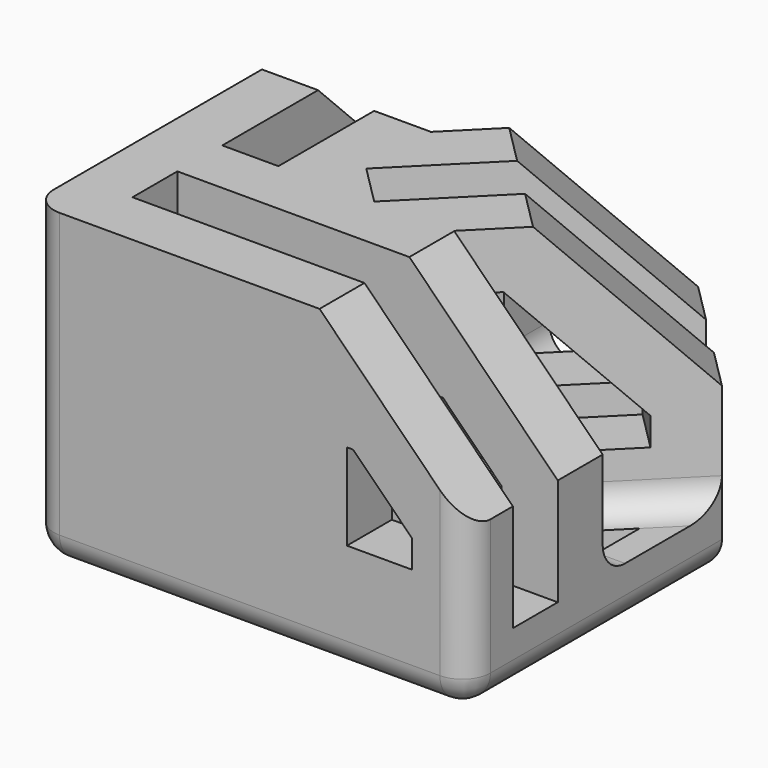
from build123d import *

# Parameters (mm, degrees)
F1_DEPTH      = 41
F3_DEPTH      = 9
F4_SIZE       = 23.8
F5_SIZE       = 23.8
F7_DEPTH      = 9
F9_DEPTH      = 28.2
F11_DEPTH     = 34.5
F13_DEPTH     = 32.2
F14_R         = 4.49999
F15_T4_DEPTH  = 56.311183182
F15_T10_DEPTH = 35.158116908
F15_T15_DEPTH = 56.311183182
F15_T21_DEPTH = 35.158116908
F15_T23_DEPTH = 61.25
F15_T25_DEPTH = 37.45
F15_T28_ANGLE = 90
F15_T30_ANGLE = 90
F15_T32_ANGLE = 90


# Not quite as in the source:
# - a fillet or chamfer that OpenCascade refuses, or shapes differently, is made with other operations: its cross-section is extruded or revolved along the edge and cut away or added
# - a fillet or chamfer is up to 0.001 mm smaller than in the source, because OpenCascade refuses the exact size


with BuildPart() as f1:
    # F0 (on Top) → F1 (new body)
    with BuildSketch(Plane.XY):
        Polygon((0, 70), (0, 0), (70, 0), (70, 9), (9, 9), (9, 18), (70, 18), (70, 27), (46.091883092, 27), (70, 50.908116908), (63.6360389693, 57.2720779386), (33.3639610307, 27), (27, 33.3639610307), (57.2720779386, 63.6360389693), (50.908116908, 70), (27, 46.091883092), (27, 70), (18, 70), (18, 27), (9, 27), (9, 70), align=None)
    extrude(amount=F1_DEPTH)

    # F2 (on face) → F3 (join)
    with BuildSketch(Plane(origin=(0, 0, 0), x_dir=(1, 0, 0), z_dir=(0, 0, -1))):
        Polygon((70, -50.908116908), (70, 0), (0, 0), (0, -70), (50.908116908, -70), align=None)
    extrude(amount=F3_DEPTH)

    # F4
    f4_edges = [f1.edges().sort_by_distance(p)[0] for p in [
        (70, 4.5, 41),
        (70, 22.5, 41),
        (22.5, 70, 41),
        (4.5, 70, 41),
    ]]
    chamfer(f4_edges, length=F4_SIZE)

    # F5
    f5_edges = [f1.edges().sort_by_distance(p)[0] for p in [
        (66.818019, 54.090097, 41),
        (54.090097, 66.818019, 41),
    ]]
    chamfer(f5_edges, length=F5_SIZE)

    # F6 (on face) → F7 (cut, through all)
    with BuildSketch(Plane.XY):
        with BuildLine():
            Line((9, 56.5), (9, 31.5))
            ThreePointArc((9, 31.5), (10.3180194847, 28.3180194847), (13.5, 27))
            ThreePointArc((13.5, 27), (16.6819805153, 28.3180194847), (18, 31.5))
            Line((18, 31.5), (18, 56.5))
            ThreePointArc((18, 56.5), (16.6819805153, 59.6819805153), (13.5, 61))
            ThreePointArc((13.5, 61), (10.3180194847, 59.6819805153), (9, 56.5))
        make_face()
        with BuildLine():
            Line((56.5, 18), (13.5, 18))
            ThreePointArc((13.5, 18), (10.3180194847, 16.6819805153), (9, 13.5))
            ThreePointArc((9, 13.5), (10.3180194847, 10.3180194847), (13.5, 9))
            Line((13.5, 9), (56.5, 9))
            ThreePointArc((56.5, 9), (59.6819805153, 10.3180194847), (61, 13.5))
            ThreePointArc((61, 13.5), (59.6819805153, 16.6819805153), (56.5, 18))
        make_face()
        with BuildLine():
            Line((47.7261363926, 54.0900974233), (30.1819805153, 36.545941546))
            ThreePointArc((30.1819805153, 36.545941546), (28.8639610307, 33.3639610307), (30.1819805153, 30.1819805153))
            ThreePointArc((30.1819805153, 30.1819805153), (33.3639610307, 28.8639610307), (36.545941546, 30.1819805153))
            Line((36.545941546, 30.1819805153), (54.0900974233, 47.7261363926))
            ThreePointArc((54.0900974233, 47.7261363926), (55.408116908, 50.908116908), (54.0900974233, 54.0900974233))
            ThreePointArc((54.0900974233, 54.0900974233), (50.908116908, 55.408116908), (47.7261363926, 54.0900974233))
        make_face()
        Polygon((40.0441558773, 65.5), (31.5, 65.5), (31.5, 56.9558441227), align=None)
        Polygon((65.5, 40.0441558773), (56.9558441227, 31.5), (65.5, 31.5), align=None)
    extrude(amount=-F7_DEPTH, mode=Mode.SUBTRACT)

    # F8 (on face) → F9 (cut)
    with BuildSketch(Plane(origin=(9.545941546, -9.545941546, 0), x_dir=(0.7071067812, 0.7071067812, 0), z_dir=(0.7071067812, -0.7071067812, 0))):
        Polygon((56.1837661841, 32), (56.1837661841, 9), (76.4949493661, 9), (76.4949493661, 13.4720779386), (57.9670273048, 32), align=None)
    extrude(amount=-F9_DEPTH, mode=Mode.SUBTRACT)

    # F10 (on face) → F11 (cut)
    with BuildSketch(Plane.YZ.offset(27)):
        Polygon((50.591883092, 22.8801948466), (50.591883092, 9), (61, 9), (61, 13.4720779386), (51.591883092, 22.8801948466), align=None)
    extrude(amount=-F11_DEPTH, mode=Mode.SUBTRACT)

    # F12 (on face) → F13 (cut)
    with BuildSketch(Plane(origin=(0, 27, 0), x_dir=(-1, 0, 0), z_dir=(0, 1, 0))):
        Polygon((-61, 13.4720779386), (-61, 9), (-50.591883092, 9), (-50.591883092, 22.8801948466), (-51.591883092, 22.8801948466), align=None)
    extrude(amount=-F13_DEPTH, mode=Mode.SUBTRACT)

    # F14 (radius 4.5 in the source; OpenCascade refuses exactly that, so slightly less here)
    f14_edges = [f1.edges().sort_by_distance(p)[0] for p in [
        (35, 0, -9),
        (70, 25.454058, -9),
        (60.454058, 60.454058, -9),
        (25.454058, 70, -9),
        (0, 35, -9),
    ]]
    fillet(f14_edges, radius=F14_R)

    # F15: fillet of radius 4.5 on 7 edges, made by hand


with BuildPart() as f15_tool2:
    # F15_s3 → F15_t4 (new body)
    with BuildSketch(Plane(origin=(28.5909902577, 28.5909902577, 0), x_dir=(0, 0, 1), z_dir=(0.7071067812, 0.7071067812, 0))):
        with BuildLine():
            ThreePointArc((4.5, 13.5), (1.3180194847, 14.8180194847), (0, 18))
            Line((0, 18), (0, 13.5))
            Line((0, 13.5), (4.5, 13.5))
        make_face()
    extrude(amount=F15_T4_DEPTH)

    split(bisect_by=Plane.YZ.offset(70), keep=Keep.BOTTOM)

    split(bisect_by=Plane.XZ.offset(-18), keep=Keep.BOTTOM)


with BuildPart() as f1_1:
    add(f1.part)

    # F15_t1: union F15_tool2
    add(f15_tool2.part)


with BuildPart() as f15_tool8:
    # F15_s9 → F15_t10 (new body)
    with BuildSketch(Plane.YZ.offset(70)):
        with BuildLine():
            ThreePointArc((27, 4.5), (28.3180194847, 1.3180194847), (31.5, 0))
            Line((31.5, 0), (27, 0))
            Line((27, 0), (27, 4.5))
        make_face()
    extrude(amount=-F15_T10_DEPTH)

    split(bisect_by=Plane(origin=(9.545941546, -9.545941546, 0), x_dir=(0, 0, 1), z_dir=(0.7071067812, -0.7071067812, 0)), keep=Keep.TOP)


with BuildPart() as f1_2:
    add(f1_1.part)

    # F15_t7: union F15_tool8
    add(f15_tool8.part)


with BuildPart() as f15_tool13:
    # F15_s14 → F15_t15 (new body)
    with BuildSketch(Plane(origin=(68.4090097423, 68.4090097423, 0), x_dir=(0, 0, 1), z_dir=(-0.7071067812, -0.7071067812, 0))):
        with BuildLine():
            ThreePointArc((4.5, 13.5), (1.3180194847, 14.8180194847), (0, 18))
            Line((0, 18), (0, 13.5))
            Line((0, 13.5), (4.5, 13.5))
        make_face()
    extrude(amount=F15_T15_DEPTH)

    split(bisect_by=Plane.XZ.offset(-70), keep=Keep.TOP)

    split(bisect_by=Plane.YZ.offset(18), keep=Keep.TOP)


with BuildPart() as f1_3:
    add(f1_2.part)

    # F15_t12: union F15_tool13
    add(f15_tool13.part)


with BuildPart() as f15_tool19:
    # F15_s20 → F15_t21 (new body)
    with BuildSketch(Plane.XZ.offset(-34.841883092)):
        with BuildLine():
            ThreePointArc((27, 4.5), (28.3180194847, 1.3180194847), (31.5, 0))
            Line((31.5, 0), (27, 0))
            Line((27, 0), (27, 4.5))
        make_face()
    extrude(amount=-F15_T21_DEPTH)

    split(bisect_by=Plane(origin=(-3.1819805153, 3.1819805153, 0), x_dir=(0, 0, 1), z_dir=(-0.7071067812, 0.7071067812, 0)), keep=Keep.TOP)


with BuildPart() as f1_4:
    add(f1_3.part)

    # F15_t18: union F15_tool19
    add(f15_tool19.part)

    # F15_s24 → F15_t23 (cut)
    with BuildSketch(Plane.XY.offset(-9)):
        with BuildLine():
            ThreePointArc((0, 4.5), (1.3180194847, 1.3180194847), (4.5, 0))
            Line((4.5, 0), (0, 0))
            Line((0, 0), (0, 4.5))
        make_face()
    extrude(amount=F15_T23_DEPTH, mode=Mode.SUBTRACT)

    # F15_s26 → F15_t25 (cut)
    with BuildSketch(Plane.XY.offset(-9)):
        with BuildLine():
            ThreePointArc((70, 4.5), (68.6819805153, 1.3180194847), (65.5, 0))
            Line((65.5, 0), (70, 0))
            Line((70, 0), (70, 4.5))
        make_face()
        with BuildLine():
            ThreePointArc((0, 65.5), (1.3180194847, 68.6819805153), (4.5, 70))
            Line((4.5, 70), (0, 70))
            Line((0, 70), (0, 65.5))
        make_face()
    extrude(amount=F15_T25_DEPTH, mode=Mode.SUBTRACT)

    # F15_s27 → F15_t28 (revolve, cut)
    with BuildSketch(Plane.XZ.offset(-65.5)):
        with BuildLine():
            ThreePointArc((4.49999, -9), (1.3180165557, -7.6819834443), (0, -4.50001))
            Line((0, -4.50001), (0, -9))
            Line((0, -9), (4.49999, -9))
        make_face()
    revolve(axis=Axis((4.5, 65.5, -9), (0, 0, -1)), revolution_arc=F15_T28_ANGLE, mode=Mode.SUBTRACT)

    # F15_s29 → F15_t30 (revolve, cut)
    with BuildSketch(Plane.XZ.offset(-4.5)):
        with BuildLine():
            ThreePointArc((65.50001, -9), (68.6819834443, -7.6819834443), (70, -4.50001))
            Line((70, -4.50001), (70, -9))
            Line((70, -9), (65.50001, -9))
        make_face()
    revolve(axis=Axis((65.5, 4.5, -9), (0, 0, -1)), revolution_arc=F15_T30_ANGLE, mode=Mode.SUBTRACT)

    # F15_s31 → F15_t32 (revolve, cut)
    with BuildSketch(Plane.YZ.offset(4.5)):
        with BuildLine():
            ThreePointArc((4.49999, -9), (1.3180165557, -7.6819834443), (0, -4.50001))
            Line((0, -4.50001), (0, -9))
            Line((0, -9), (4.49999, -9))
        make_face()
    revolve(axis=Axis((4.5, 4.5, -9), (0, 0, -1)), revolution_arc=F15_T32_ANGLE, mode=Mode.SUBTRACT)


solid = f1_4.part
